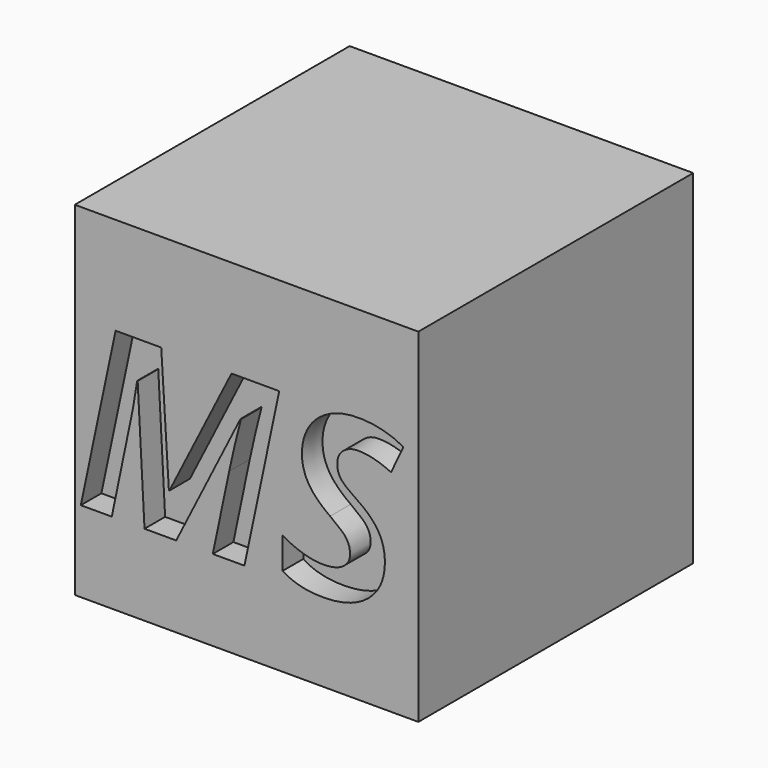
from build123d import *

# Parameters (mm, degrees)
F0_W          = 40
F0_H          = 40
F1_DEPTH      = 40
F2_R          = 5
F3_DEPTH      = 10
F4_R          = 5
F5_DEPTH      = 10
F6_R          = 5
F7_DEPTH      = 9.9
F8_R          = 5
F9_DEPTH      = 9.9
F10_TEXT_SIZE = 26.9048870205
F11_DEPTH     = 3


# Not quite as in the source:
# - Text() gives the source's letters only with a copy of the font that has no kerning and outlines rounded to 1/6400 em; it was checked with that copy


with BuildPart() as f1:
    # F0 (on Front) → F1 (new body)
    with BuildSketch(Plane.XZ):
        with Locations((20, -20)):
            Rectangle(F0_W, F0_H)
    extrude(amount=F1_DEPTH)

    # F2 (on Right) → F3 (join)
    with BuildSketch(Plane.YZ):
        with Locations((-20, -20)):
            Circle(F2_R)
    extrude(amount=-F3_DEPTH)

    # F4 (on Right) → F5 (join)
    with BuildSketch(Plane.YZ):
        with Locations((-20, -20)):
            Circle(F4_R)
    extrude(amount=-F5_DEPTH)

    # F6 (on Right) → F7 (join)
    with BuildSketch(Plane.YZ):
        with Locations((-20, -20)):
            Circle(F6_R)
    extrude(amount=-F7_DEPTH)

    # F8 (on face) → F9 (join)
    with BuildSketch(Plane(origin=(0, 0, -40), x_dir=(1, 0, 0), z_dir=(0, 0, -1))):
        with Locations((20, 20)):
            Circle(F8_R)
    extrude(amount=F9_DEPTH)

    # F10 (on face) → F11 (cut)
    with BuildSketch(Plane.XZ.offset(40)):
        with Locations((0, -30.5699127956)):
            Text('MS', F10_TEXT_SIZE, font='Open Sans', font_style=FontStyle.BOLDITALIC, text_align=(TextAlign.LEFT, TextAlign.BOTTOM))
    extrude(amount=-F11_DEPTH, mode=Mode.SUBTRACT)


solid = f1.part
